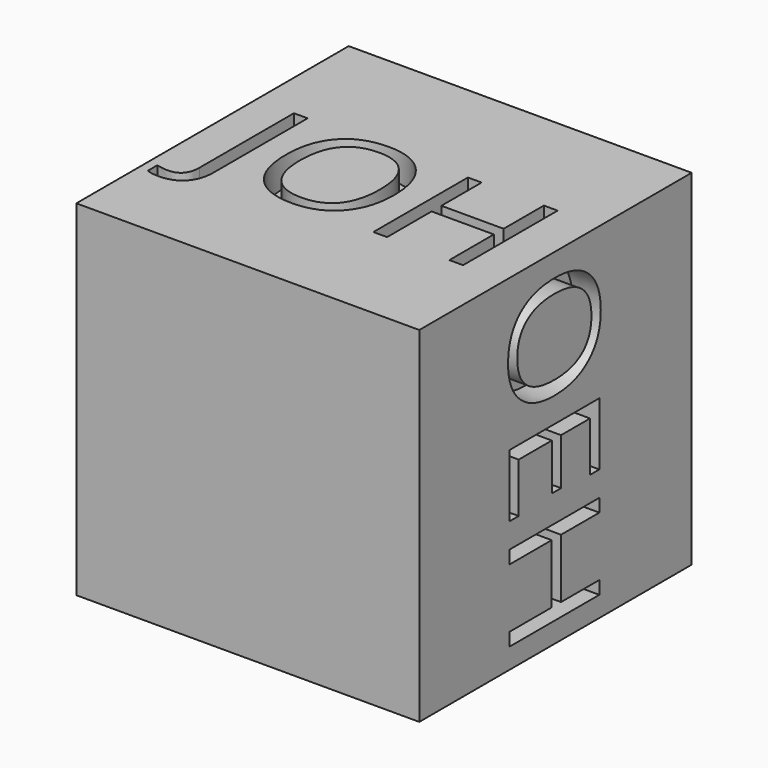
from build123d import *

# Parameters (mm, degrees)
F0_W         = 153.5039333152
F0_H         = 152.4
F1_DEPTH     = 154.432
F2_TEXT_SIZE = 74.0833373533
F3_DEPTH     = 12.7
F4_TEXT_SIZE = 70.5555555556
F5_DEPTH     = 12.7
F6_TEXT_SIZE = 69.8886915214
F7_DEPTH     = 12.7
F8_TEXT_SIZE = 70.5555555556
F9_DEPTH     = 12.7


# Not quite as in the source:
# - Text() gives the source's letters only with a copy of the font that has no kerning and outlines rounded to 1/6400 em; it was checked with that copy


with BuildPart() as f1:
    # F0 (on Top) → F1 (new body)
    with BuildSketch(Plane.XY):
        with Locations((-76.7519666576, 76.2)):
            Rectangle(F0_W, F0_H)
    extrude(amount=F1_DEPTH)

    # F2 (on face) → F3 (cut)
    with BuildSketch(Plane.XY.offset(154.432)):
        with Locations((-143.6014734209, 47.8722080588)):
            Text('JOH', F2_TEXT_SIZE, font='Open Sans', text_align=(TextAlign.LEFT, TextAlign.BOTTOM))
    extrude(amount=-F3_DEPTH, mode=Mode.SUBTRACT)

    # F4 (on face) → F5 (cut)
    with BuildSketch(Plane.YZ):
        with Locations(Location((50.3736776431, 148.475488185), (0, 0, -90))):
            Text('OEH', F4_TEXT_SIZE, font='Open Sans', text_align=(TextAlign.LEFT, TextAlign.BOTTOM))
    extrude(amount=-F5_DEPTH, mode=Mode.SUBTRACT)

    # F6 (on face) → F7 (cut)
    with BuildSketch(Plane(origin=(0, 0, 0), x_dir=(1, 0, 0), z_dir=(0, 0, -1))):
        with Locations(Location((-7.8821498707, -53.2627105713), (0, 0, -180))):
            Text('KRH', F6_TEXT_SIZE, font='Open Sans', text_align=(TextAlign.LEFT, TextAlign.BOTTOM))
    extrude(amount=-F7_DEPTH, mode=Mode.SUBTRACT)

    # F8 (on face) → F9 (cut)
    with BuildSketch(Plane(origin=(-153.5039333152, 0, 0), x_dir=(0, -1, 0), z_dir=(-1, 0, 0))):
        with Locations(Location((-45.4528046114, -0.9789886038), (0, 0, 90))):
            Text('ORH', F8_TEXT_SIZE, font='Open Sans', text_align=(TextAlign.LEFT, TextAlign.BOTTOM))
    extrude(amount=-F9_DEPTH, mode=Mode.SUBTRACT)


solid = f1.part
